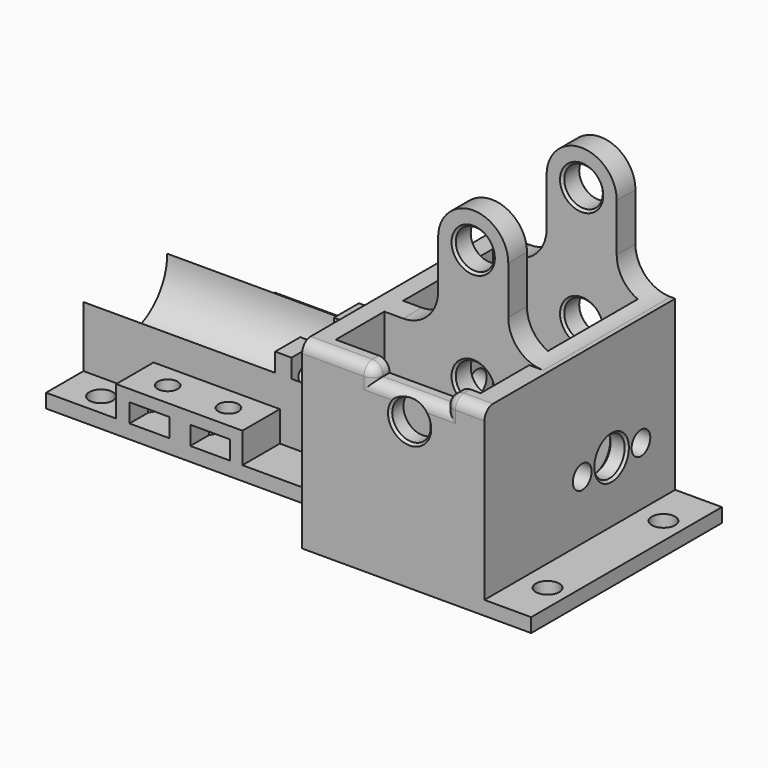
from build123d import *

# Parameters (mm, degrees)
F0_W          = 39
F0_H          = 51
F0_W_2        = 31
F0_H_2        = 13
F0_H_3        = 24
F0_W_3        = 10
F0_R          = 2.5
F1_DEPTH      = 3
F2_DEPTH      = 36
F3_R          = 4.125
F4_DEPTH      = 49.001
F5_W          = 15
F5_H          = 5
F6_DEPTH      = 25.25
F7_R          = 4.125
F8_DEPTH      = 51.001
F3_W          = 10
F3_H          = 3
F3_W_2        = 5.8
F3_W_3        = 4.2
F9_DEPTH      = 65
F10_W         = 3.5
F10_H         = 6.7
F11_DEPTH     = 20
F12_R         = 1.5
F13_DEPTH     = 4
F5_H_2        = 4
F14_DEPTH     = 2.5
F15_R         = 2.5
F16_DEPTH     = 3.001
F15_R_2       = 2.15
F17_DEPTH     = 6.5
F18_DEPTH     = 4
F19_R         = 2.5
F19_R_2       = 1.5
F20_DEPTH     = 69.501
F21_SIZE      = 0.5
F22_T1_DEPTH  = 18.95
F22_T3_DEPTH  = 11.95
F22_T5_DEPTH  = 0.2
F22_T7_DEPTH  = 15
F22_T9_DEPTH  = 7.45
F22_S13_W     = 2.3
F22_S13_H     = 2.3
F22_T14_DEPTH = 2.3
F22_S19_W     = 2.3
F22_S19_H     = 2.3
F22_T20_DEPTH = 2.3
F22_T27_DEPTH = 5.95
F22_T31_DEPTH = 20.75
F22_T38_DEPTH = 20.75
F22_T42_DEPTH = 5.95
F23_T1_DEPTH  = 5
F23_T3_DEPTH  = 5
F23_T8_DEPTH  = 42.5
F23_T14_DEPTH = 23.75
F23_T16_DEPTH = 42.5
F23_T18_DEPTH = 42.5


# Not quite as in the source:
# - a fillet or chamfer that OpenCascade refuses, or shapes differently, is made with other operations: its cross-section is extruded or revolved along the edge and cut away or added
# - a feature names something its author has since deleted; it is built from what else it names


with BuildPart() as f1:
    # F0 (on Top) → F1 (new body)
    with BuildSketch(Plane.XY):
        with Locations((19.5, 0)):
            Rectangle(F0_W, F0_H)
        with Locations((19.5, -15)):
            Rectangle(F0_W_2, F0_H_2, mode=Mode.SUBTRACT)
        with Locations((19.5, 8.5)):
            Rectangle(F0_W_2, F0_H_3, mode=Mode.SUBTRACT)
        with Locations((19.5, 8.5)):
            Rectangle(F0_W_2, F0_H_3)
        with Locations((44, 0)):
            Rectangle(F0_W_3, F0_H)
        with Locations((44.5, -15.5)):
            Circle(F0_R, mode=Mode.SUBTRACT)
        with Locations((44.5, 15.5)):
            Circle(F0_R, mode=Mode.SUBTRACT)
        with Locations((19.5, -15)):
            Rectangle(F0_W_2, F0_H_2)
    extrude(amount=-F1_DEPTH)

    # F0 (on Top) → F2 (join)
    with BuildSketch(Plane.XY):
        with Locations((19.5, 0)):
            Rectangle(F0_W, F0_H)
        with Locations((19.5, -15)):
            Rectangle(F0_W_2, F0_H_2, mode=Mode.SUBTRACT)
        with Locations((19.5, 8.5)):
            Rectangle(F0_W_2, F0_H_3, mode=Mode.SUBTRACT)
    extrude(amount=F2_DEPTH)

    # F3 (on face) → F4 (cut, through all)
    with BuildSketch(Plane(origin=(0, 0, 0), x_dir=(0, -1, 0), z_dir=(-1, 0, 0))):
        with Locations((-8.5, 13)):
            Circle(F3_R)
    extrude(amount=-F4_DEPTH, mode=Mode.SUBTRACT)

    # F5 (on face) → F6 (join)
    with BuildSketch(Plane.XY.offset(36)):
        with Locations((23, 23)):
            Rectangle(F5_W, F5_H)
        with Locations((23, -6)):
            Rectangle(F5_W, F5_H)
    extrude(amount=F6_DEPTH)

    # F7 (on face) → F8 (cut, through all)
    with BuildSketch(Plane(origin=(0, 25.5, 0), x_dir=(-1, 0, 0), z_dir=(0, 1, 0))):
        with Locations((-23, 28.5)):
            Circle(F7_R)
        with Locations((-23, 53.75)):
            Circle(F7_R)
    extrude(amount=-F8_DEPTH, mode=Mode.SUBTRACT)

    # F3 (on face) → F9 (join)
    with BuildSketch(Plane(origin=(0, 0, 0), x_dir=(0, -1, 0), z_dir=(-1, 0, 0))):
        with BuildLine():
            Line((-19.7, 0), (-19.7, -3))
            Line((-19.7, -3), (2.7, -3))
            Line((2.7, -3), (2.7, 0))
            Line((2.7, 0), (2.7, 13))
            ThreePointArc((2.7, 13), (-8.5, 1.8), (-19.7, 13))
            Line((-19.7, 13), (-19.7, 0))
        make_face()
        with Locations((7.7, -1.5)):
            Rectangle(F3_W, F3_H)
        with Locations((-22.6, -1.5)):
            Rectangle(F3_W_2, F3_H)
        with Locations((-27.6, -1.5)):
            Rectangle(F3_W_3, F3_H)
    extrude(amount=F9_DEPTH)

    # F10 (on face) → F11 (join)
    with BuildSketch(Plane(origin=(0, 0, -3), x_dir=(1, 0, 0), z_dir=(0, 0, -1))):
        with Locations((-22.25, -0.65)):
            Rectangle(F10_W, F10_H)
        with Locations((-22.25, -16.35)):
            Rectangle(F10_W, F10_H)
    extrude(amount=-F11_DEPTH)

    # F12 (on face) → F13 (cut)
    with BuildSketch(Plane(origin=(-24, 0, 0), x_dir=(0, -1, 0), z_dir=(-1, 0, 0))):
        with Locations((-16.35, 12.55)):
            Circle(F12_R)
        with Locations((-0.65, 12.55)):
            Circle(F12_R)
    extrude(amount=-F13_DEPTH, mode=Mode.SUBTRACT)

    # F5 (on face) → F14 (cut)
    with BuildSketch(Plane.XY.offset(36)):
        with Locations((23, -23.5)):
            Rectangle(F5_W, F5_H_2)
    extrude(amount=-F14_DEPTH, mode=Mode.SUBTRACT)

    # F15 (on face) → F16 (cut, through all)
    with BuildSketch(Plane.XY):
        with Locations((-57, -8)):
            Circle(F15_R)
        with Locations((-10, -8)):
            Circle(F15_R)
        with Locations((-10, 25)):
            Circle(F15_R)
        with Locations((-57, 25)):
            Circle(F15_R)
    extrude(amount=-F16_DEPTH, mode=Mode.SUBTRACT)

    # F15 (on face) → F17 (join)
    with BuildSketch(Plane.XY):
        Polygon((-34.1569219382, -7.7), (-32.0784609691, -4.1), (-27.9215390309, -4.1), (-25.617175976, -8.0912738902), (-25.617175976, -12.7), (-23, -12.7), (-23, -2.7), (-50, -2.7), (-50, -12.7), (-47.1569219382, -12.7), (-47.1569219382, -7.7), (-45.0784609691, -4.1), (-40.9215390309, -4.1), (-38.617175976, -8.0912738902), (-38.617175976, -12.7), (-34.1569219382, -12.7), align=None)
        Polygon((-38.8430780618, 29.7), (-38.8430780618, 24.7), (-40.9215390309, 21.1), (-45.0784609691, 21.1), (-47.1569219382, 24.7), (-47.1569219382, 29.7), (-50, 29.7), (-50, 19.7), (-23, 19.7), (-23, 29.7), (-25.8430780618, 29.7), (-25.8430780618, 24.7), (-27.9215390309, 21.1), (-32.0784609691, 21.1), (-34.1569219382, 24.7), (-34.1569219382, 29.7), align=None)
        Polygon((-47.1569219382, -12.7), (-38.617175976, -12.7), (-38.617175976, -8.0912738902), (-40.9215390309, -4.1), (-45.0784609691, -4.1), (-47.1569219382, -7.7), align=None)
        with Locations((-43, -7.7)):
            Circle(F15_R_2, mode=Mode.SUBTRACT)
        Polygon((-27.9215390309, -4.1), (-32.0784609691, -4.1), (-34.1569219382, -7.7), (-34.1569219382, -12.7), (-25.617175976, -12.7), (-25.617175976, -8.0912738902), align=None)
        with Locations((-30, -7.7)):
            Circle(F15_R_2, mode=Mode.SUBTRACT)
        Polygon((-40.9215390309, 21.1), (-38.8430780618, 24.7), (-38.8430780618, 29.7), (-47.1569219382, 29.7), (-47.1569219382, 24.7), (-45.0784609691, 21.1), align=None)
        with Locations((-43, 24.7)):
            Circle(F15_R_2, mode=Mode.SUBTRACT)
        Polygon((-25.8430780618, 29.7), (-34.1569219382, 29.7), (-34.1569219382, 24.7), (-32.0784609691, 21.1), (-27.9215390309, 21.1), (-25.8430780618, 24.7), align=None)
        with Locations((-30, 24.7)):
            Circle(F15_R_2, mode=Mode.SUBTRACT)
    extrude(amount=F17_DEPTH)

    # F15 (on face) → F18 (cut)
    with BuildSketch(Plane.XY):
        Polygon((-47.1569219382, -12.7), (-38.617175976, -12.7), (-38.617175976, -8.0912738902), (-40.9215390309, -4.1), (-45.0784609691, -4.1), (-47.1569219382, -7.7), align=None)
        with Locations((-43, -7.7)):
            Circle(F15_R_2, mode=Mode.SUBTRACT)
        Polygon((-27.9215390309, -4.1), (-32.0784609691, -4.1), (-34.1569219382, -7.7), (-34.1569219382, -12.7), (-25.617175976, -12.7), (-25.617175976, -8.0912738902), align=None)
        with Locations((-30, -7.7)):
            Circle(F15_R_2, mode=Mode.SUBTRACT)
        Polygon((-40.9215390309, 21.1), (-38.8430780618, 24.7), (-38.8430780618, 29.7), (-47.1569219382, 29.7), (-47.1569219382, 24.7), (-45.0784609691, 21.1), align=None)
        with Locations((-43, 24.7)):
            Circle(F15_R_2, mode=Mode.SUBTRACT)
        Polygon((-25.8430780618, 29.7), (-34.1569219382, 29.7), (-34.1569219382, 24.7), (-32.0784609691, 21.1), (-27.9215390309, 21.1), (-25.8430780618, 24.7), align=None)
        with Locations((-30, 24.7)):
            Circle(F15_R_2, mode=Mode.SUBTRACT)
    extrude(amount=F18_DEPTH, mode=Mode.SUBTRACT)

    # F19 (on face) → F20 (cut, through all)
    with BuildSketch(Plane.YZ.offset(-20.5)):
        with Locations((0.65, 12.55)):
            Circle(F19_R)
        with Locations((16.35, 12.55)):
            Circle(F19_R)
        with Locations((16.35, 12.55)):
            Circle(F19_R_2, mode=Mode.SUBTRACT)
        with Locations((16.35, 12.55)):
            Circle(F19_R_2)
    extrude(amount=F20_DEPTH, mode=Mode.SUBTRACT)

    # F21
    f21_edges = [f1.edges().sort_by_distance(p)[0] for p in [
        (27.125, -8.5, 28.5),
        (39, 12.625, 13),
        (27.125, 20.5, 28.5),
        (4, 12.625, 13),
        (27.125, -3.5, 28.5),
        (27.125, -3.5, 53.75),
        (27.125, -21.5, 28.5),
        (27.125, 25.5, 53.75),
        (27.125, 25.5, 28.5),
        (27.125, -8.5, 53.75),
        (27.125, 20.5, 53.75),
        (0, 12.625, 13),
        (35, 12.625, 13),
        (27.125, -25.5, 28.5),
    ]]
    chamfer(f21_edges, length=F21_SIZE)

    # F22: fillet of radius 2.3 on 7 edges, made by hand

    # F22_s2 → F22_t1 (cut)
    with BuildSketch(Plane.YZ.offset(-5.75)):
        with BuildLine():
            ThreePointArc((-25.5, 33.7), (-24.8263455967, 35.3263455967), (-23.2, 36))
            Line((-23.2, 36), (-25.5, 36))
            Line((-25.5, 36), (-25.5, 33.7))
        make_face()
    extrude(amount=F22_T1_DEPTH, mode=Mode.SUBTRACT)

    # F22_s4 → F22_t3 (cut)
    with BuildSketch(Plane.YZ.offset(32.8)):
        with BuildLine():
            ThreePointArc((-25.5, 33.7), (-24.8263455967, 35.3263455967), (-23.2, 36))
            Line((-23.2, 36), (-25.5, 36))
            Line((-25.5, 36), (-25.5, 33.7))
        make_face()
    extrude(amount=F22_T3_DEPTH, mode=Mode.SUBTRACT)

    # F22_s6 → F22_t5 (cut)
    with BuildSketch(Plane.XY.offset(33.5)):
        with BuildLine():
            ThreePointArc((13.2, -25.5), (14.8263455967, -24.8263455967), (15.5, -23.2))
            Line((15.5, -23.2), (15.5, -25.5))
            Line((15.5, -25.5), (13.2, -25.5))
        make_face()
        with BuildLine():
            ThreePointArc((32.8, -25.5), (31.1736544033, -24.8263455967), (30.5, -23.2))
            Line((30.5, -23.2), (30.5, -25.5))
            Line((30.5, -25.5), (32.8, -25.5))
        make_face()
    extrude(amount=F22_T5_DEPTH, mode=Mode.SUBTRACT)

    # F22_s8 → F22_t7 (cut)
    with BuildSketch(Plane.YZ.offset(15.5)):
        with BuildLine():
            ThreePointArc((-25.5, 31.2), (-24.8263455967, 32.8263455967), (-23.2, 33.5))
            Line((-23.2, 33.5), (-25.5, 33.5))
            Line((-25.5, 33.5), (-25.5, 31.2))
        make_face()
    extrude(amount=F22_T7_DEPTH, mode=Mode.SUBTRACT)

    # F22_s10 → F22_t9 (cut)
    with BuildSketch(Plane.XZ.offset(15.75)):
        with BuildLine():
            ThreePointArc((13.2, 36), (14.8263455967, 35.3263455967), (15.5, 33.7))
            Line((15.5, 33.7), (15.5, 36))
            Line((15.5, 36), (13.2, 36))
        make_face()
        with BuildLine():
            ThreePointArc((30.5, 33.7), (31.1736544033, 35.3263455967), (32.8, 36))
            Line((32.8, 36), (30.5, 36))
            Line((30.5, 36), (30.5, 33.7))
        make_face()
    extrude(amount=F22_T9_DEPTH, mode=Mode.SUBTRACT)


with BuildPart() as f22_tool12:
    # F22_s13 → F22_t14 (new body)
    with BuildSketch(Plane.XZ.offset(23.2)):
        with Locations((14.35, 34.85)):
            Rectangle(F22_S13_W, F22_S13_H)
    extrude(amount=F22_T14_DEPTH)

    # F22_s15 → F22_t16 (revolve, cut)
    with BuildSketch(Plane(origin=(13.2, -23.2, 33.7), x_dir=(-0.7071067812, 0, -0.7071067812), z_dir=(-0.7071067812, 0, 0.7071067812))):
        with BuildLine():
            ThreePointArc((0, -2.3), (2.3, 0), (0, 2.3))
            Line((0, 2.3), (0, -2.3))
        make_face()
    revolve(axis=Axis((13.2, -23.2, 33.7), (0, -1, 0)), mode=Mode.SUBTRACT)


with BuildPart() as f1_1:
    add(f1.part)

    # F22_t11: cut F22_tool12
    add(f22_tool12.part, mode=Mode.SUBTRACT)


with BuildPart() as f22_tool18:
    # F22_s19 → F22_t20 (new body)
    with BuildSketch(Plane.YZ.offset(32.8)):
        with Locations((-24.35, 34.85)):
            Rectangle(F22_S19_W, F22_S19_H)
    extrude(amount=-F22_T20_DEPTH)

    # F22_s21 → F22_t22 (revolve, cut)
    with BuildSketch(Plane(origin=(32.8, -23.2, 33.7), x_dir=(0, 0.7071067812, -0.7071067812), z_dir=(0, 0.7071067812, 0.7071067812))):
        with BuildLine():
            ThreePointArc((0, -2.3), (2.3, 0), (0, 2.3))
            Line((0, 2.3), (0, -2.3))
        make_face()
    revolve(axis=Axis((32.8, -23.2, 33.7), (-1, 0, 0)), mode=Mode.SUBTRACT)


with BuildPart() as f1_2:
    add(f1_1.part)

    # F22_t17: cut F22_tool18
    add(f22_tool18.part, mode=Mode.SUBTRACT)


with BuildPart() as f22_tool25:
    # F22_s26 → F22_t27 (new body)
    with BuildSketch(Plane.XY.offset(33.7)):
        with BuildLine():
            ThreePointArc((13.2, -25.5), (14.8263455967, -24.8263455967), (15.5, -23.2))
            Line((15.5, -23.2), (15.5, -25.5))
            Line((15.5, -25.5), (13.2, -25.5))
        make_face()
    extrude(amount=-F22_T27_DEPTH)

    split(bisect_by=Plane.XY.offset(33.5), keep=Keep.BOTTOM)


with BuildPart() as f22_tool29:
    # F22_s30 → F22_t31 (new body)
    with BuildSketch(Plane.YZ.offset(9.75)):
        with BuildLine():
            ThreePointArc((-25.5, 31.2), (-24.8263455967, 32.8263455967), (-23.2, 33.5))
            Line((-23.2, 33.5), (-25.5, 33.5))
            Line((-25.5, 33.5), (-25.5, 31.2))
        make_face()
    extrude(amount=F22_T31_DEPTH)

    split(bisect_by=Plane.YZ.offset(15.5), keep=Keep.BOTTOM)


with BuildPart() as f22_tool25_1:
    add(f22_tool25.part)

    # F22_t33: intersect F22_tool29
    add(f22_tool29.part, mode=Mode.INTERSECT)


with BuildPart() as f1_3:
    add(f1_2.part)

    # F22_t23: cut F22_tool25
    add(f22_tool25_1.part, mode=Mode.SUBTRACT)


with BuildPart() as f22_tool36:
    # F22_s37 → F22_t38 (new body)
    with BuildSketch(Plane.YZ.offset(15.5)):
        with BuildLine():
            ThreePointArc((-25.5, 31.2), (-24.8263455967, 32.8263455967), (-23.2, 33.5))
            Line((-23.2, 33.5), (-25.5, 33.5))
            Line((-25.5, 33.5), (-25.5, 31.2))
        make_face()
    extrude(amount=F22_T38_DEPTH)

    split(bisect_by=Plane.YZ.offset(30.5), keep=Keep.TOP)


with BuildPart() as f22_tool40:
    # F22_s41 → F22_t42 (new body)
    with BuildSketch(Plane.XY.offset(33.7)):
        with BuildLine():
            ThreePointArc((32.8, -25.5), (31.1736544033, -24.8263455967), (30.5, -23.2))
            Line((30.5, -23.2), (30.5, -25.5))
            Line((30.5, -25.5), (32.8, -25.5))
        make_face()
    extrude(amount=-F22_T42_DEPTH)

    split(bisect_by=Plane.XY.offset(33.5), keep=Keep.BOTTOM)


with BuildPart() as f22_tool36_1:
    add(f22_tool36.part)

    # F22_t44: intersect F22_tool40
    add(f22_tool40.part, mode=Mode.INTERSECT)


with BuildPart() as f1_4:
    add(f1_3.part)

    # F22_t34: cut F22_tool36
    add(f22_tool36_1.part, mode=Mode.SUBTRACT)

    # F23: fillet of radius 7.5 on 8 edges, made by hand

    # F23_s2 → F23_t1 (join)
    with BuildSketch(Plane.XZ.offset(3.5)):
        with BuildLine():
            ThreePointArc((15.5, 43.5), (13.3033008589, 38.1966991411), (8, 36))
            Line((8, 36), (15.5, 36))
            Line((15.5, 36), (15.5, 43.5))
        make_face()
        with BuildLine():
            ThreePointArc((38, 36), (32.6966991411, 38.1966991411), (30.5, 43.5))
            Line((30.5, 43.5), (30.5, 36))
            Line((30.5, 36), (38, 36))
        make_face()
    extrude(amount=F23_T1_DEPTH)

    # F23_s4 → F23_t3 (join)
    with BuildSketch(Plane.XZ.offset(-25.5)):
        with BuildLine():
            ThreePointArc((15.5, 43.5), (13.3033008589, 38.1966991411), (8, 36))
            Line((8, 36), (15.5, 36))
            Line((15.5, 36), (15.5, 43.5))
        make_face()
        with BuildLine():
            ThreePointArc((30.5, 43.5), (32.6966991411, 38.1966991411), (38, 36))
            Line((38, 36), (30.5, 36))
            Line((30.5, 36), (30.5, 43.5))
        make_face()
    extrude(amount=F23_T3_DEPTH)


with BuildPart() as f23_tool6:
    # F23_s7 → F23_t8 (new body)
    with BuildSketch(Plane.XZ.offset(27.25)):
        with BuildLine():
            ThreePointArc((38, 36), (32.6966991411, 38.1966991411), (30.5, 43.5))
            Line((30.5, 43.5), (30.5, 36))
            Line((30.5, 36), (38, 36))
        make_face()
    extrude(amount=-F23_T8_DEPTH)

    split(bisect_by=Plane.YZ.offset(35), keep=Keep.TOP)

    split(bisect_by=Plane.XZ.offset(3.5), keep=Keep.BOTTOM)


with BuildPart() as f1_5:
    add(f1_4.part)

    # F23_t5: union F23_tool6
    add(f23_tool6.part)


with BuildPart() as f23_tool12:
    # F23_s13 → F23_t14 (new body)
    with BuildSketch(Plane.XZ.offset(-1.75)):
        with BuildLine():
            ThreePointArc((30.5, 43.5), (32.6966991411, 38.1966991411), (38, 36))
            Line((38, 36), (30.5, 36))
            Line((30.5, 36), (30.5, 43.5))
        make_face()
    extrude(amount=-F23_T14_DEPTH)

    split(bisect_by=Plane.YZ.offset(35), keep=Keep.TOP)


with BuildPart() as f1_6:
    add(f1_5.part)

    # F23_t11: union F23_tool12
    add(f23_tool12.part)

    # F23_s17 → F23_t16 (cut)
    with BuildSketch(Plane.XZ.offset(-44.25)):
        with BuildLine():
            ThreePointArc((23, 61.25), (17.6966991411, 59.0533008589), (15.5, 53.75))
            Line((15.5, 53.75), (15.5, 61.25))
            Line((15.5, 61.25), (23, 61.25))
        make_face()
        with BuildLine():
            ThreePointArc((30.5, 53.75), (28.3033008589, 59.0533008589), (23, 61.25))
            Line((23, 61.25), (30.5, 61.25))
            Line((30.5, 61.25), (30.5, 53.75))
        make_face()
    extrude(amount=F23_T16_DEPTH, mode=Mode.SUBTRACT)

    # F23_s19 → F23_t18 (cut)
    with BuildSketch(Plane.XZ.offset(-15.25)):
        with BuildLine():
            ThreePointArc((30.5, 53.75), (28.3033008589, 59.0533008589), (23, 61.25))
            Line((23, 61.25), (30.5, 61.25))
            Line((30.5, 61.25), (30.5, 53.75))
        make_face()
        with BuildLine():
            ThreePointArc((23, 61.25), (17.6966991411, 59.0533008589), (15.5, 53.75))
            Line((15.5, 53.75), (15.5, 61.25))
            Line((15.5, 61.25), (23, 61.25))
        make_face()
    extrude(amount=F23_T18_DEPTH, mode=Mode.SUBTRACT)


solid = f1_6.part
